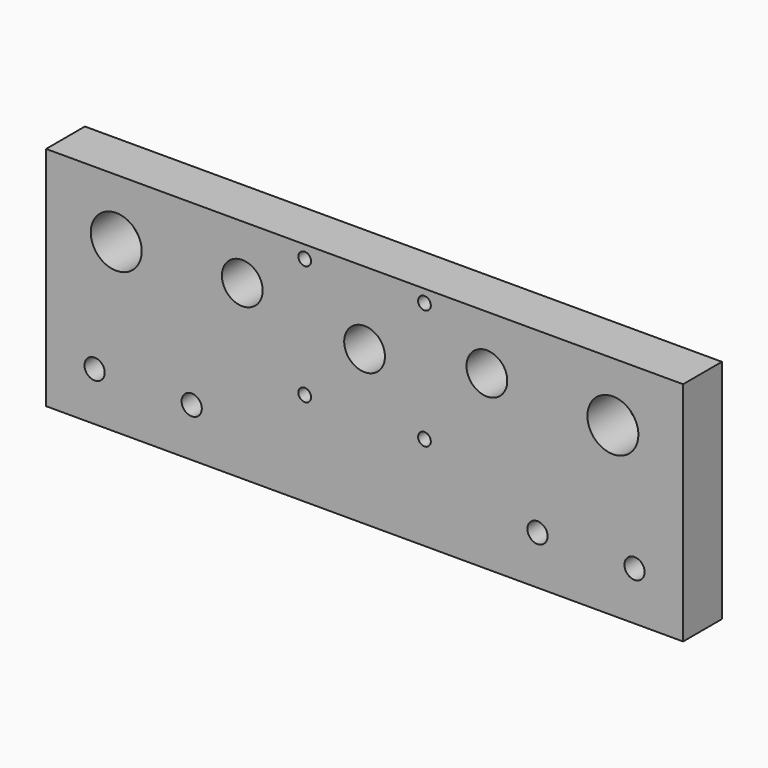
from build123d import *

# Parameters (mm, degrees)
F0_W     = 250
F0_H     = 88.9
F1_DEPTH = 9.525
F2_R     = 8
F2_R_2   = 2.5
F2_R_3   = 10
F2_R_4   = 3.96875
F3_DEPTH = 25.4


# Not quite as in the source:
# - a pattern or mirror of a feature is missing from the dataset's text; its kind, count and spacing are read off the source's solid


with BuildPart() as f1:
    # F0 (on Front) → F1 (new body, symmetric)
    with BuildSketch(Plane.XZ):
        Rectangle(F0_W, F0_H)
    extrude(amount=F1_DEPTH, both=True)

    # F2 (on face) → F3 (cut)
    with BuildSketch(Plane.XZ.offset(9.525)):
        with Locations((-48, 23.14)):
            Circle(F2_R)
        with Locations((0, 15.95)):
            Circle(F2_R)
        with Locations((-23.5, -7.55)):
            Circle(F2_R_2)
        with Locations((-23.5, 39.45)):
            Circle(F2_R_2)
        with Locations((-97.455, 21.3)):
            Circle(F2_R_3)
        with Locations((-67.85, -25.4)):
            Circle(F2_R_4)
        with Locations((-105.95, -25.4)):
            Circle(F2_R_4)
    f3 = extrude(amount=-F3_DEPTH, mode=Mode.SUBTRACT)

    # F3_copies: F3 across plane
    add(f3.mirror(Plane(origin=(0, 0, 0), x_dir=(0, 0, 1), z_dir=(1, 0, 0))), mode=Mode.SUBTRACT)


solid = f1.part
